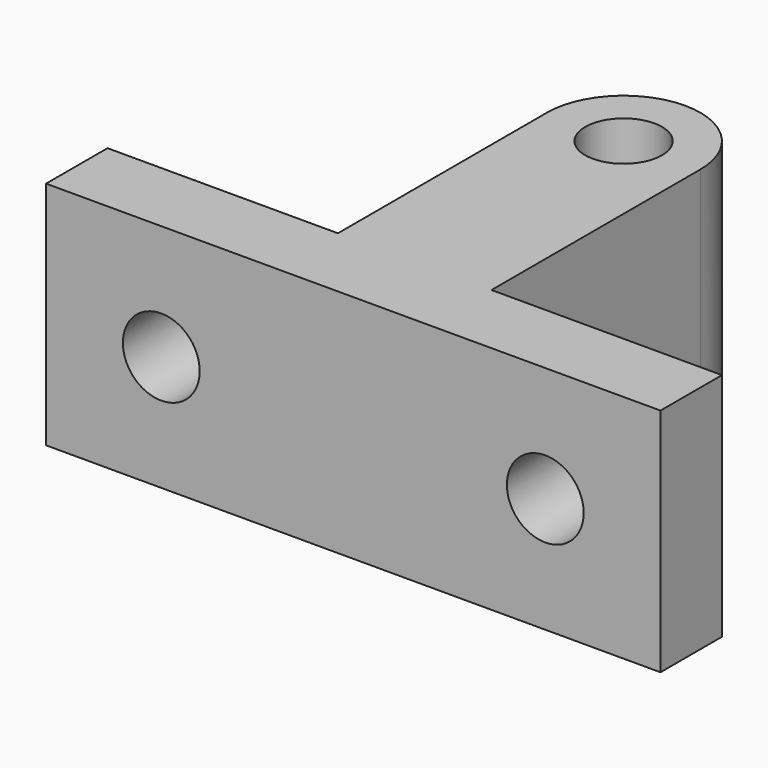
from build123d import *

# Parameters (mm, degrees)
F0_R     = 1.5875
F1_DEPTH = 9.525
F3_D     = 3.175
F5_D     = 3.175


# Not quite as in the source:
# - a length typed as a fraction of an inch, garbled in the dataset ("3 / 203.2 mm" for 3/8 in), is restored


with BuildPart() as f1:
    # F0 (on Top) → F1 (new body)
    with BuildSketch(Plane.XY):
        with BuildLine():
            Line((1.6785456881, 9.5886874095), (1.6785456881, -1.2063125905))
            Line((1.6785456881, -1.2063125905), (8.0285456881, -1.2063125905))
            Line((8.0285456881, -1.2063125905), (8.0285456881, 9.5886874095))
            ThreePointArc((8.0285456881, 9.5886874095), (7.0986097184, 11.8337514397), (4.8535456881, 12.7636874095))
            ThreePointArc((4.8535456881, 12.7636874095), (2.6084816578, 11.8337514397), (1.6785456881, 9.5886874095))
        make_face()
        with Locations((4.8535456881, 9.5886874095)):
            Circle(F0_R, mode=Mode.SUBTRACT)
        Polygon((-7.8464543119, -1.2063125905), (-7.8464543119, -4.3813125905), (17.5535456881, -4.3813125905), (17.5535456881, -1.2063125905), (8.0285456881, -1.2063125905), (1.6785456881, -1.2063125905), align=None)
    extrude(amount=F1_DEPTH)

    # F3 (through all)
    with Locations(Plane(origin=(0, -1.2063125905, 0), x_dir=(-1, 0, 0), z_dir=(0, 1, 0))):
        with Locations((-12.7910456881, 4.7625)):
            Hole(F3_D / 2)

    # F5 (through all)
    with Locations(Plane(origin=(0, -1.2063125905, 0), x_dir=(-1, 0, 0), z_dir=(0, 1, 0))):
        with Locations((3.0839543119, 4.7625)):
            Hole(F5_D / 2)


solid = f1.part
